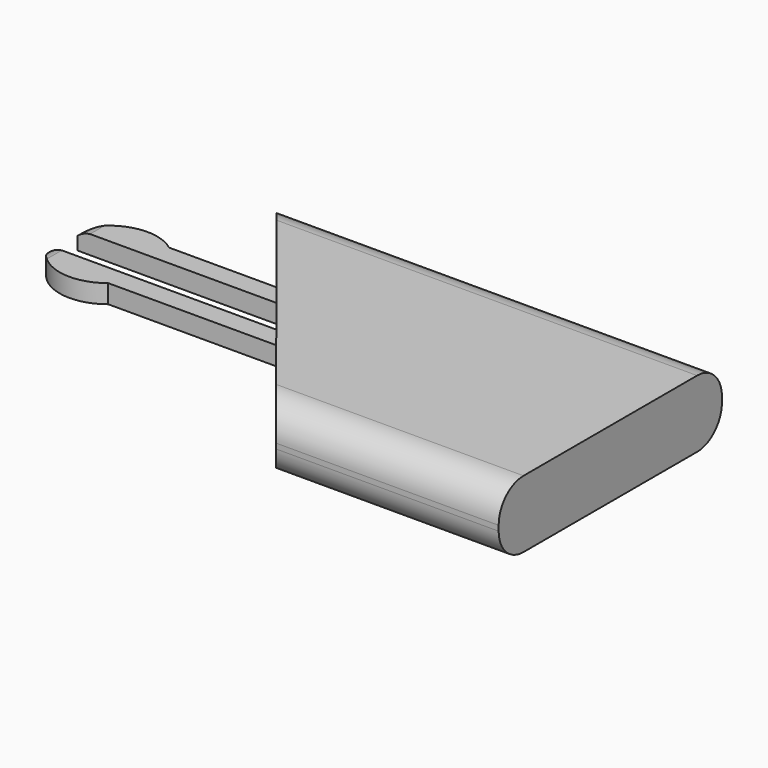
from build123d import *

# Parameters (mm, degrees)
F2_DEPTH  = 3.5
F4_DEPTH  = 1
F6_DEPTH  = 1.8
F8_DEPTH  = 1.2
F9_R      = 3
F11_DEPTH = 17.1864665007


with BuildPart() as f2:
    # F1 (on Top) → F2 (new body)
    with BuildSketch(Plane.XY):
        Polygon((48.5598316574, 13.5), (5.4801683426, 13.5), (27.0198316574, -13.5), align=None)
        Polygon((48.5598316574, 13.5), (27.0198316574, -13.5), (48.5598316574, -13.5), align=None)
    extrude(amount=-F2_DEPTH)

    # F3 (on Top) → F4 (cut)
    with BuildSketch(Plane.XY):
        Polygon((44.7943471372, 11.7882982132), (6.8457046456, 11.7882982132), (25.8198775993, -11.9958558036), align=None)
    extrude(amount=-F4_DEPTH, mode=Mode.SUBTRACT)

    # F5 (on face) → F6 (join)
    with BuildSketch(Plane.XY):
        with BuildLine():
            ThreePointArc((2.8793278964, 3.7278809202), (3.7658696299, 2.8294612951), (4.3820146982, 1.7278809202))
            Line((4.3820146982, 1.7278809202), (14.8715565456, 1.7278809202))
            Line((14.8715565456, 1.7278809202), (17.594606702, -1.6854665007))
            Line((17.594606702, -1.6854665007), (4.3985029231, -1.6854665007))
            ThreePointArc((4.3985029231, -1.6854665007), (3.7999051439, -2.783585132), (2.9334215452, -3.6854665007))
            Line((2.9334215452, -3.6854665007), (19.1901373179, -3.6854665007))
            Line((19.1901373179, -3.6854665007), (25.8198775993, -11.9958558036))
            Line((25.8198775993, -11.9958558036), (44.7943471372, 11.7882982132))
            Line((44.7943471372, 11.7882982132), (6.8457046456, 11.7882982132))
            Line((6.8457046456, 11.7882982132), (13.2760259297, 3.7278809202))
            Line((13.2760259297, 3.7278809202), (2.8793278964, 3.7278809202))
        make_face()
        Polygon((5.4801683426, 13.5), (6.8457046456, 11.7882982132), (44.7943471372, 11.7882982132), (25.8198775993, -11.9958558036), (27.0198316574, -13.5), (48.5598316574, 13.5), align=None)
        with BuildLine():
            Line((-4.3820146982, 1.7278809202), (4.3820146982, 1.7278809202))
            ThreePointArc((4.3820146982, 1.7278809202), (3.7658696299, 2.8294612951), (2.8793278964, 3.7278809202))
            ThreePointArc((2.8793278964, 3.7278809202), (-1.2508065023, 4.5412672663), (-4.3820146982, 1.7278809202))
        make_face()
        with BuildLine():
            ThreePointArc((2.9334215452, -3.6854665007), (3.7999051439, -2.783585132), (4.3985029231, -1.6854665007))
            Line((4.3985029231, -1.6854665007), (-4.3985029231, -1.6854665007))
            ThreePointArc((-4.3985029231, -1.6854665007), (-1.2396031062, -4.5443381728), (2.9334215452, -3.6854665007))
        make_face()
        Polygon((48.5598316574, 13.5), (27.0198316574, -13.5), (48.5598316574, -13.5), align=None)
    extrude(amount=F6_DEPTH)

    # F7 (on face) → F8 (join)
    with BuildSketch(Plane.XY.offset(1.8)):
        Polygon((48.5598316574, 13.5), (5.4801683426, 13.5), (13.2760259297, 3.7278809202), (14.8715565456, 1.7278809202), (17.594606702, -1.6854665007), (19.1901373179, -3.6854665007), (27.0198316574, -13.5), (48.5598316574, -13.5), align=None)
    extrude(amount=F8_DEPTH)

    # F9
    f9_edges = [f2.edges().sort_by_distance(p)[0] for p in [
        (27.02, 13.5, 3),
        (27.02, 13.5, -3.5),
        (37.789832, -13.5, 3),
        (37.789832, -13.5, -3.5),
    ]]
    fillet(f9_edges, radius=F9_R)

    # F10 (on face) → F11 (cut, through all)
    with BuildSketch(Plane.XZ.offset(3.6854665007)):
        with BuildLine():
            ThreePointArc((-4.430251196, 1.1966986349), (-3.7397455906, 1.6462971281), (-2.9335320779, 1.8164634239))
            Line((-2.9335320779, 1.8164634239), (-4.430251196, 1.8164634239))
            Line((-4.430251196, 1.8164634239), (-4.430251196, 1.1966986349))
        make_face()
    extrude(amount=-F11_DEPTH, mode=Mode.SUBTRACT)


solid = f2.part
